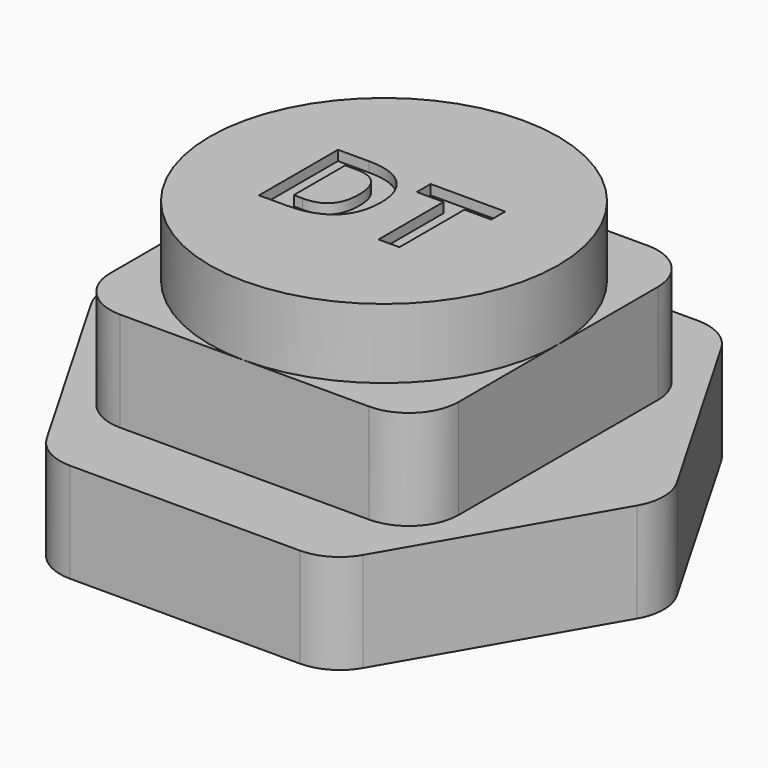
from build123d import *

# Parameters (mm, degrees)
F1_DEPTH     = 10
F2_W         = 35
F2_H         = 35
F3_DEPTH     = 10
F4_R         = 5
F5_R         = 17.5
F6_DEPTH     = 7
F7_TEXT_SIZE = 13.8888888889
F8_DEPTH     = 1


# Not quite as in the source:
# - Text() gives the source's letters only with a copy of the font that has no kerning and outlines rounded to 1/6400 em; it was checked with that copy


with BuildPart() as f1:
    # F0 (on Top) → F1 (new body)
    with BuildSketch(Plane.XY):
        Polygon((14.4337567297, 25), (-14.4337567297, 25), (-28.8675134595, 0), (-14.4337567297, -25), (14.4337567297, -25), (28.8675134595, 0), align=None)
    extrude(amount=F1_DEPTH)

    # F2 (on face) → F3 (join)
    with BuildSketch(Plane.XY.offset(10)):
        Rectangle(F2_W, F2_H)
    extrude(amount=F3_DEPTH)

    # F4
    f4_edges = [f1.edges().sort_by_distance(p)[0] for p in [
        (-28.867513, 0, 5),
        (-14.433757, -25, 5),
        (14.433757, -25, 5),
        (28.867513, 0, 5),
        (14.433757, 25, 5),
        (-14.433757, 25, 5),
        (-17.5, 17.5, 15),
        (-17.5, -17.5, 15),
        (17.5, -17.5, 15),
        (17.5, 17.5, 15),
    ]]
    fillet(f4_edges, radius=F4_R)

    # F5 (on face) → F6 (join)
    with BuildSketch(Plane.XY.offset(20)):
        Circle(F5_R)
    extrude(amount=F6_DEPTH)

    # F7 (on face) → F8 (cut)
    with BuildSketch(Plane.XY.offset(27)):
        with Locations((-9.5, -5.3806644273)):
            Text('DT', F7_TEXT_SIZE, font='Open Sans', font_style=FontStyle.BOLD, text_align=(TextAlign.LEFT, TextAlign.BOTTOM))
    extrude(amount=-F8_DEPTH, mode=Mode.SUBTRACT)


solid = f1.part
